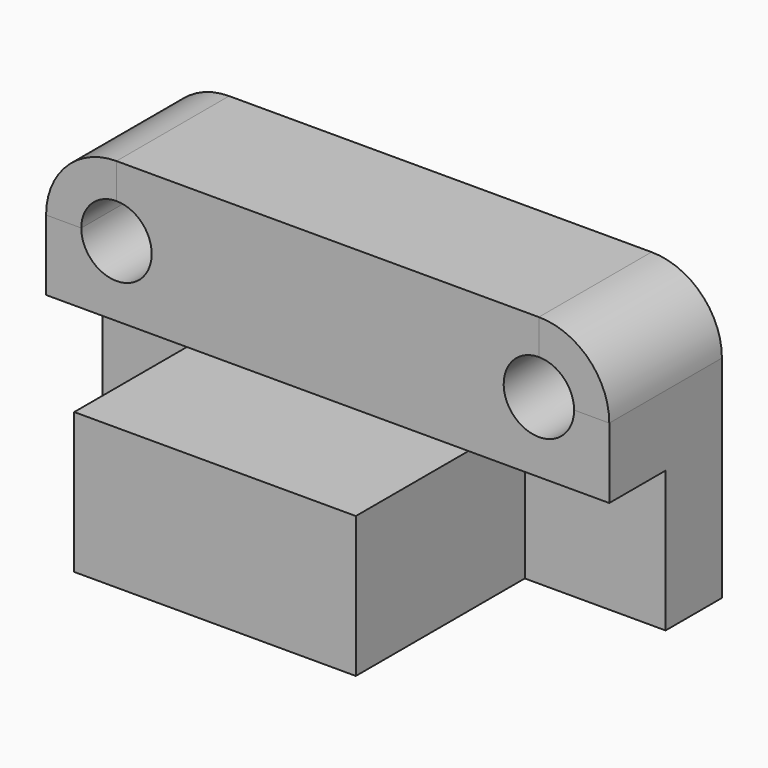
from build123d import *

# Parameters (mm, degrees)
F0_W     = 101.6
F0_H     = 50.8
F1_DEPTH = 101.6
F0_W_2   = 50.8
F2_DEPTH = 25.4
F3_DEPTH = 50.8
F4_DEPTH = 50.8
F5_R     = 25.39999
F5_2_R   = 25.39999


# Not quite as in the source:
# - a fillet or chamfer is up to 0.001 mm smaller than in the source, because OpenCascade refuses the exact size


with BuildPart() as f1:
    # F0 (on Front) → F1 (new body)
    with BuildSketch(Plane.XZ):
        with Locations((-101.6, 25.4)):
            Rectangle(F0_W, F0_H)
    extrude(amount=F1_DEPTH)

    # F0 (on Front) → F2 (join)
    with BuildSketch(Plane.XZ):
        with Locations((-177.8, 25.4)):
            Rectangle(F0_W_2, F0_H)
        with Locations((-25.4, 25.4)):
            Rectangle(F0_W_2, F0_H)
    extrude(amount=F2_DEPTH)

    # F0 (on Front) → F3 (join)
    with BuildSketch(Plane.XZ):
        with BuildLine():
            Line((-50.8, 50.8), (0, 50.8))
            Line((0, 50.8), (0, 76.2))
            Line((0, 76.2), (-12.7, 76.2))
            ThreePointArc((-12.7, 76.2), (-34.3802561211, 67.2197438789), (-25.4, 88.9))
            Line((-25.4, 88.9), (-25.4, 101.6))
            Line((-25.4, 101.6), (-177.8, 101.6))
            Line((-177.8, 101.6), (-177.8, 88.9))
            ThreePointArc((-177.8, 88.9), (-168.8197438789, 85.1802561211), (-165.1, 76.2))
            ThreePointArc((-165.1, 76.2), (-177.8, 63.5), (-190.5, 76.2))
            Line((-190.5, 76.2), (-203.2, 76.2))
            Line((-203.2, 76.2), (-203.2, 50.8))
            Line((-203.2, 50.8), (-152.4, 50.8))
            Line((-152.4, 50.8), (-50.8, 50.8))
        make_face()
    extrude(amount=F3_DEPTH)


with BuildPart() as f4:
    # F0 (on Front) → F4 (new body)
    with BuildSketch(Plane.XZ):
        with BuildLine():
            Line((-12.7, 76.2), (0, 76.2))
            Line((0, 76.2), (0, 101.6))
            Line((0, 101.6), (-25.4, 101.6))
            Line((-25.4, 101.6), (-25.4, 88.9))
            ThreePointArc((-25.4, 88.9), (-16.4197438789, 85.1802561211), (-12.7, 76.2))
        make_face()
    extrude(amount=F4_DEPTH)

    # F5 (radius 25.4 in the source; OpenCascade refuses exactly that, so slightly less here)
    f5_edges = [f4.edges().sort_by_distance(p)[0] for p in [
        (0, -25.4, 101.6),
    ]]
    fillet(f5_edges, radius=F5_R)


with BuildPart() as f4b:
    # F0 (on Front) → F4, piece 2 (new body)
    with BuildSketch(Plane.XZ):
        with BuildLine():
            Line((-203.2, 101.6), (-203.2, 76.2))
            Line((-203.2, 76.2), (-190.5, 76.2))
            ThreePointArc((-190.5, 76.2), (-186.7802561211, 85.1802561211), (-177.8, 88.9))
            Line((-177.8, 88.9), (-177.8, 101.6))
            Line((-177.8, 101.6), (-203.2, 101.6))
        make_face()
    extrude(amount=F4_DEPTH)

    # F5#2 (radius 25.4 in the source; OpenCascade refuses exactly that, so slightly less here)
    f5_2_edges = [f4b.edges().sort_by_distance(p)[0] for p in [
        (-203.2, -25.4, 101.6),
    ]]
    fillet(f5_2_edges, radius=F5_2_R)


solid = Compound([f1.part, f4.part, f4b.part])
